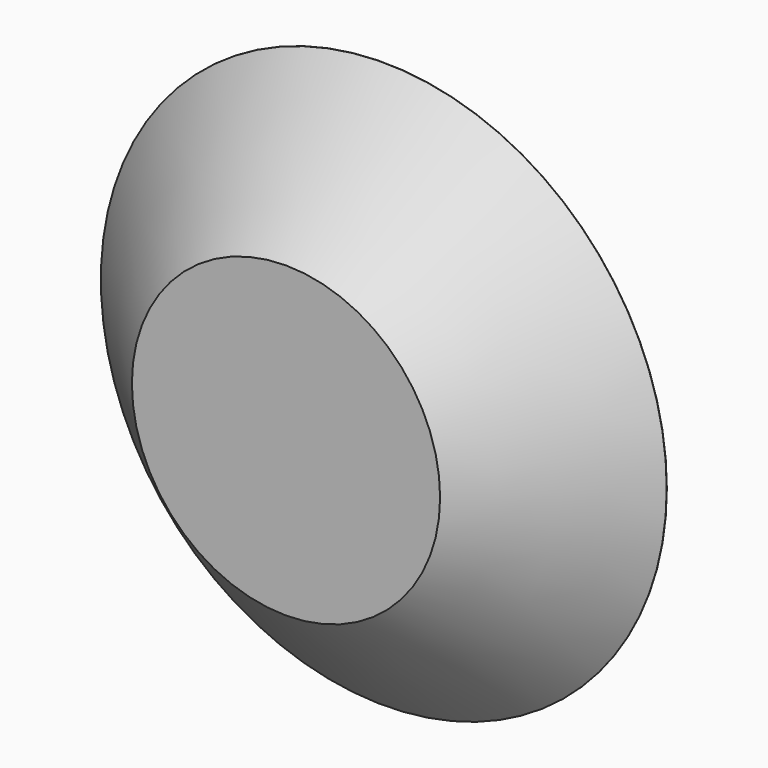
from build123d import *

# Parameters (mm, degrees)
F0_R     = 57.3756528728
F1_DEPTH = 25.4
F1_TAPER = -3


# Not quite as in the source:
# - a fillet or chamfer that OpenCascade refuses, or shapes differently, is made with other operations: its cross-section is extruded or revolved along the edge and cut away or added


with BuildPart() as f1:
    # F0 (on Front) → F1 (new body)
    with BuildSketch(Plane.XZ):
        Circle(F0_R)
    extrude(amount=-F1_DEPTH, taper=F1_TAPER)

    # F2: chamfer of 25.4 on 1 edges, made by hand

    # F2_s1 → F2_t2 (revolve, cut)
    with BuildSketch(Plane.XY):
        Polygon((58.7049861613, 25.3651901828), (31.9756528728, 0), (57.3756528728, 0), align=None)
    revolve(axis=Axis((0, 0, 0), (0, 1, 0)), mode=Mode.SUBTRACT)


solid = f1.part
